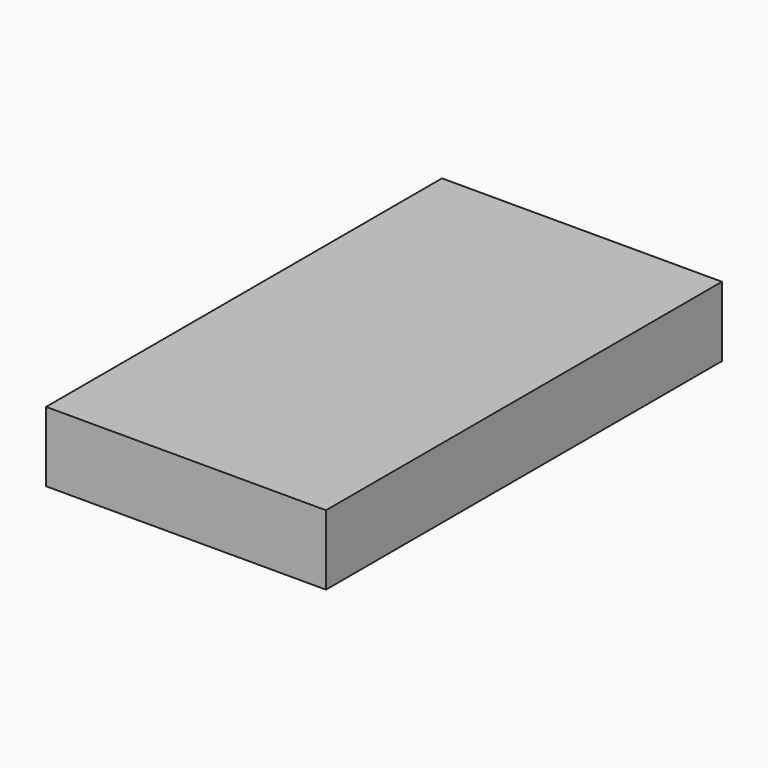
from build123d import *

# Parameters (mm, degrees)
F0_W     = 81.3410878181
F0_H     = 143.805667758
F0_W_2   = 72.0662102103
F0_H_2   = 133.9904665947
F1_DEPTH = 20.3194860369
F2_W     = 81.3410878181
F2_H     = 20.3194860369
F3_DEPTH = 139.7007852793


# Not quite as in the source:
# - the program builds the solid bodies; features that only make, move or delete a surface that nothing else refers to are left out


with BuildPart() as f1:
    # F0 (on Top) → F1 (new body)
    with BuildSketch(Plane.XY):
        Rectangle(F0_W, F0_H)
        Rectangle(F0_W_2, F0_H_2, mode=Mode.SUBTRACT)
    extrude(amount=-F1_DEPTH)

    # F2 (on face) → F3 (join)
    with BuildSketch(Plane.XZ.offset(71.902833879)):
        with Locations((0, -10.1597430184)):
            Rectangle(F2_W, F2_H)
    extrude(amount=-F3_DEPTH)


solid = f1.part
